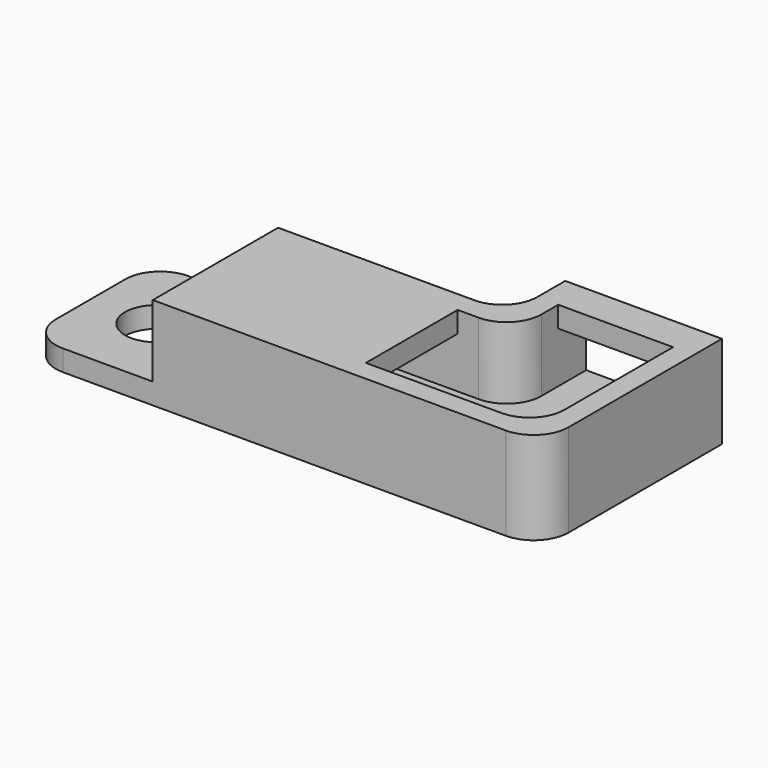
from build123d import *

# Parameters (mm, degrees)
F0_W     = 33.12
F0_H     = 22.44
F1_DEPTH = 13.28
F0_W_2   = 17.88
F0_R     = 4.5
F2_DEPTH = 3
F3_T     = -3
F4_W     = 8
F4_H     = 16.44
F5_DEPTH = 3
F6_R     = 5


# Not quite as in the source:
# - a shell that OpenCascade refuses in one call is made with other operations: the cavity is built on its own and cut out
# - a feature names something its author has since deleted; it is built from what else it names


with BuildPart() as f1:
    # F0 (on Top) → F1 (new body)
    with BuildSketch(Plane.XY):
        Polygon((30.6844967631, 22.44), (30.6844967631, 0), (53.1244967631, 0), (53.1244967631, 32.44), (30.6844967631, 32.44), align=None)
        with Locations((14.1244967631, 11.22)):
            Rectangle(F0_W, F0_H)
    extrude(amount=F1_DEPTH)

    # F0 (on Top) → F2 (join)
    with BuildSketch(Plane.XY):
        with Locations((-11.3755032369, 11.22)):
            Rectangle(F0_W_2, F0_H)
        with Locations((-10.8755032369, 11.22)):
            Circle(F0_R, mode=Mode.SUBTRACT)
    extrude(amount=F2_DEPTH)

    # F3: a shell. OpenCascade refuses it in one call, so the cavity is built on its own and cut out:
    # the body offset inwards by the wall thickness, plus a prism from it out through each open face.
    f3_core = offset(f1.part, amount=F3_T, kind=Kind.INTERSECTION, mode=Mode.PRIVATE)
    f3_exits = [f3_core.faces().sort_by_distance(p)[0] for p in [
        (0.564497, 11.22, 6.64),
        (41.904497, 29.44, 6.64),
    ]]
    add(f3_core, mode=Mode.SUBTRACT)
    extrude(f3_exits, amount=-F3_T, mode=Mode.SUBTRACT)

    # F4 (on face) → F5 (cut)
    with BuildSketch(Plane.XY.offset(13.28)):
        with Locations((29.6844967631, 11.22)):
            Rectangle(F4_W, F4_H)
        Polygon((50.1244967631, 27.44), (33.6844967631, 27.44), (33.6844967631, 19.44), (33.6844967631, 3), (50.1244967631, 3), align=None)
    extrude(amount=-F5_DEPTH, mode=Mode.SUBTRACT)

    # F6
    f6_edges = [f1.edges().sort_by_distance(p)[0] for p in [
        (53.124497, 0, 6.64),
        (30.684497, 22.44, 6.64),
        (33.684497, 19.44, 8.14),
        (50.124497, 3, 8.14),
        (-20.315503, 22.44, 1.5),
        (-20.315503, 0, 1.5),
    ]]
    fillet(f6_edges, radius=F6_R)


solid = f1.part
